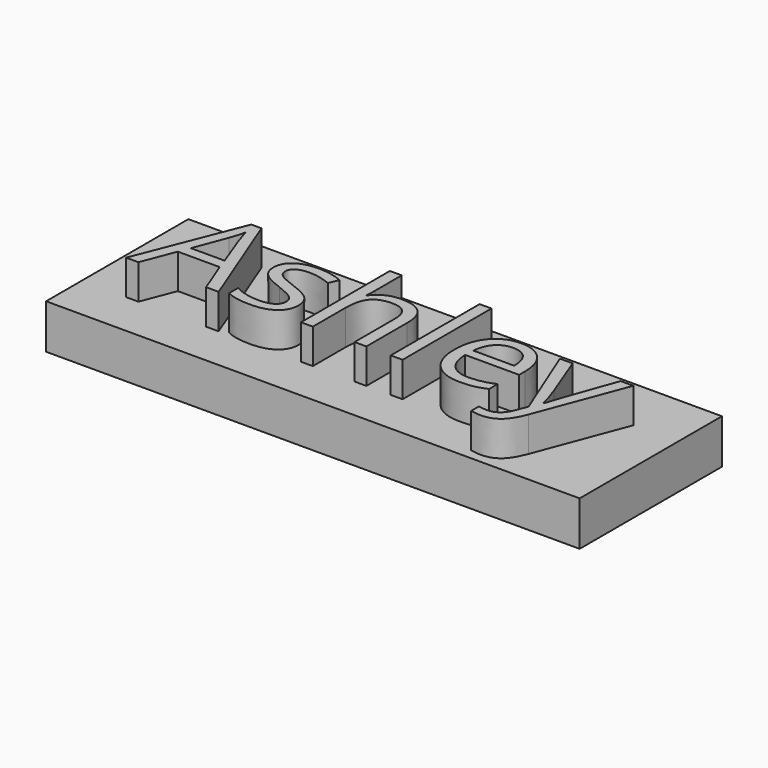
from build123d import *

# Parameters (mm, degrees)
F0_W         = 60
F0_H         = 20
F1_DEPTH     = 5
F2_TEXT_SIZE = 16.443987667
F3_DEPTH     = 8.90917


# Not quite as in the source:
# - Text() gives the source's letters only with a copy of the font that has no kerning and outlines rounded to 1/6400 em; it was checked with that copy


with BuildPart() as f1:
    # F0 (on Top) → F1 (new body)
    with BuildSketch(Plane.XY):
        Rectangle(F0_W, F0_H)
    extrude(amount=F1_DEPTH)

    # F2 (on Top) → F3 (join)
    with BuildSketch(Plane.XY):
        with Locations((-25, -5)):
            Text('Ashley', F2_TEXT_SIZE, font='Open Sans', text_align=(TextAlign.LEFT, TextAlign.BOTTOM))
    extrude(amount=F3_DEPTH)


solid = f1.part
